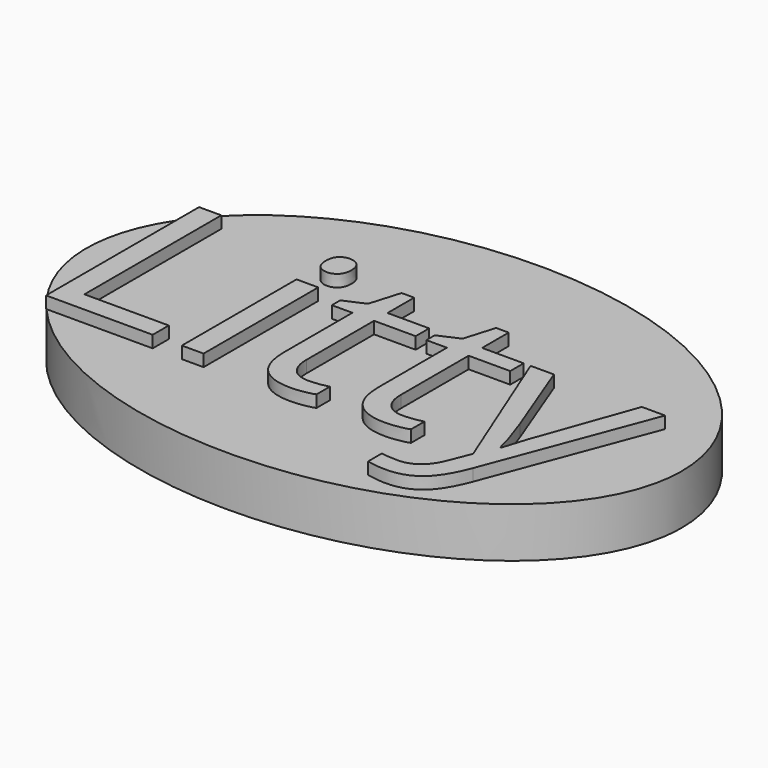
from build123d import *

# Parameters (mm, degrees)
F1_DEPTH     = 6.35
F2_TEXT_SIZE = 34.0954993164
F3_DEPTH     = 1.524


# Not quite as in the source:
# - Text() gives the source's letters only with a copy of the font that has no kerning and outlines rounded to 1/6400 em; it was checked with that copy


with BuildPart() as f1:
    # F0 (on Top) → F1 (new body)
    with BuildSketch(Plane.XY):
        with BuildLine():
            add(Edge.make_bspline(
                [(38.0976516619, -0.4230104558), (38.586102063, 43.5683684292), (-18.8046006304, 22.2071946704), (-76.1953033239, 0.8460209116), (-19.2930510315, -21.7841842146), (37.6092012609, -44.4143893408), (38.0976516619, -0.4230104558)],
                knots=[0, 0, 0, 2.0943951024, 2.0943951024, 4.1887902048, 4.1887902048, 6.2831853072, 6.2831853072, 6.2831853072], degree=2, weights=[1, 0.5, 1, 0.5, 1, 0.5, 1]))
        make_face()
    extrude(amount=F1_DEPTH)

    # F2 (on face) → F3 (join)
    with BuildSketch(Plane.XY.offset(6.35)):
        with Locations((-36.396706912, -12.4801205834)):
            Text('Litty', F2_TEXT_SIZE, font='Open Sans', text_align=(TextAlign.LEFT, TextAlign.BOTTOM))
    extrude(amount=F3_DEPTH)


solid = f1.part
